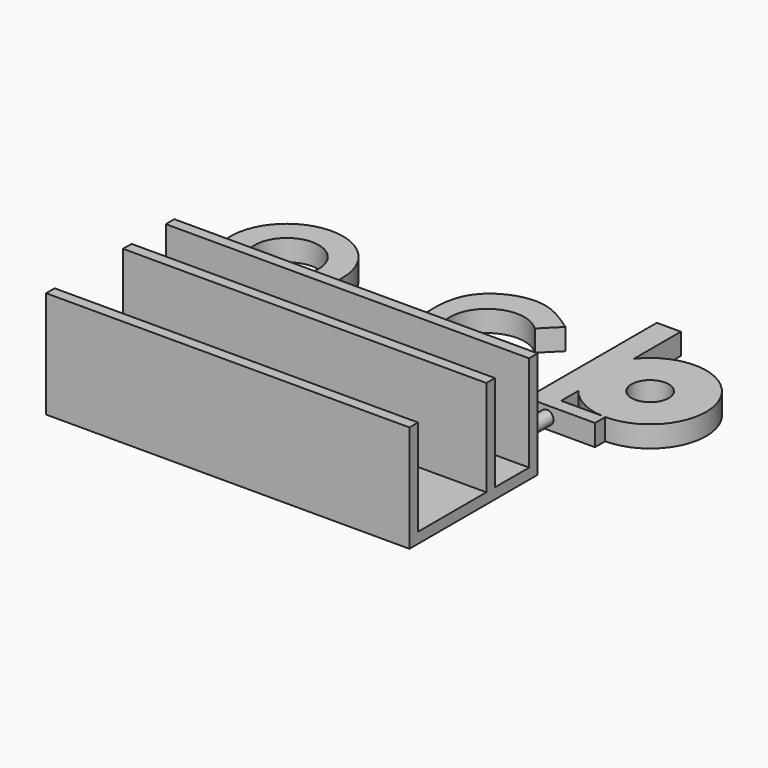
from build123d import *

# Parameters (mm, degrees)
F1_R      = 6
F2_DEPTH  = 4
F1_R_2    = 3.5
F0_R      = 7
F3_DEPTH  = 25
F5_DEPTH  = 4
F6_R      = 1.2123195681
F6_R_2    = 1.1427466474
F6_R_3    = 1.2541450495
F7_DEPTH  = 10
F9_W      = 68
F9_H      = 30
F10_DEPTH = 20
F11_W     = 68
F11_H     = 8
F11_H_2   = 16
F12_DEPTH = 18
F13_R     = 1.26
F14_DEPTH = 25


with BuildPart() as f2:
    # F1 (on Top) → F2 (new body)
    with BuildSketch(Plane.XY):
        with BuildLine():
            ThreePointArc((6, -8.6168439698), (9.3072552345, -4.8605555238), (10.5, 0))
            ThreePointArc((10.5, 0), (-9.3072552345, 4.8605555238), (6, -8.6168439698))
        make_face()
        Circle(F1_R, mode=Mode.SUBTRACT)
        with BuildLine():
            Line((10.5, -10.5), (10.5, 0))
            ThreePointArc((10.5, 0), (9.3072552345, -4.8605555238), (6, -8.6168439698))
            Line((6, -8.6168439698), (6, -10.5))
            Line((6, -10.5), (10.5, -10.5))
        make_face()
    extrude(amount=F2_DEPTH)



with BuildPart() as f2b:
    # F1 (on Top) → F2, piece 2 (new body)
    with BuildSketch(Plane.XY):
        with BuildLine():
            ThreePointArc((32.75, -5.1417409503), (40.3062430401, -6.4128776692), (44.5, 0))
            ThreePointArc((44.5, 0), (43.9671567276, 2.6787840266), (42.4497474683, 4.9497474683))
            ThreePointArc((42.4497474683, 4.9497474683), (32.4532674542, 4.8508237044), (32.75, -5.1417409503))
        make_face()
        with BuildLine():
            ThreePointArc((32.75, -5.1417409503), (32.4532674542, 4.8508237044), (42.4497474683, 4.9497474683))
            Line((42.4497474683, 4.9497474683), (45.6317279836, 8.1317279836))
            add(Edge.make_bspline(
                [(28.25, -10.5), (27.0400886154, -3.8399480871), (24.8960722969, 7.9619575442), (37.8802140743, 13.5938400363), (43.1156627298, 9.9046758889), (45.6317279836, 8.1317279836)],
                knots=[0, 0, 0, 0, 0.4021935112, 0.7127046345, 1, 1, 1, 1], degree=3))
            Line((28.25, -10.5), (32.75, -10.5))
            Line((32.75, -10.5), (32.75, -5.1417409503))
        make_face()
    extrude(amount=F2_DEPTH)

    # F0 (on Top) → F3 (cut)
    with BuildSketch(Plane.XY):
        with Locations((37.5, 0)):
            Circle(F0_R)
    extrude(amount=F3_DEPTH, mode=Mode.SUBTRACT)


with BuildPart() as f2c:
    # F1 (on Top) → F2, piece 3 (new body)
    with BuildSketch(Plane.XY):
        with BuildLine():
            Line((55.25, 17.5), (55.25, -10.5))
            Line((55.25, -10.5), (59.75, -10.5))
            Line((59.75, -10.5), (59.75, -6.4951905284))
            ThreePointArc((59.75, -6.4951905284), (57.5, 0), (59.75, 6.4951905284))
            Line((59.75, 6.4951905284), (59.75, 17.5))
            Line((59.75, 17.5), (55.25, 17.5))
        make_face()
        with BuildLine():
            ThreePointArc((59.75, 6.4951905284), (57.5, 0), (59.75, -6.4951905284))
            Line((59.75, -6.4951905284), (59.75, 6.4951905284))
        make_face()
        with BuildLine():
            Line((59.75, 6.4951905284), (59.75, -6.4951905284))
            ThreePointArc((59.75, -6.4951905284), (71.4369317712, -9.9215674165), (78.5, 0))
            ThreePointArc((78.5, 0), (71.4369317712, 9.9215674165), (59.75, 6.4951905284))
        make_face()
        with Locations((68, 0)):
            Circle(F1_R_2, mode=Mode.SUBTRACT)
    extrude(amount=F2_DEPTH)


with BuildPart() as f2_1:
    add(f2.part)

    add(f2b.part)  # F5 merges F2b

    add(f2c.part)  # F5 merges F2c
    # F4 (on Top) → F5 (join)
    with BuildSketch(Plane.XY):
        Polygon((28.25, -10.5), (10.5, -10.5), (6, -10.5), (0, -10.5), (0, -12.9), (68, -12.9), (68, -10.5), (59.75, -10.5), (55.25, -10.5), (32.75, -10.5), align=None)
        with BuildLine():
            Line((6, -10.5), (10.5, -10.5))
            Line((10.5, -10.5), (28.25, -10.5))
            Line((28.25, -10.5), (32.75, -10.5))
            Line((32.75, -10.5), (55.25, -10.5))
            Line((55.25, -10.5), (59.75, -10.5))
            Line((59.75, -10.5), (68, -10.5))
            ThreePointArc((68, -10.5), (67.7708712153, -10.4974997023), (67.5418515524, -10.49))
            Line((67.5418515524, -10.49), (0.4581484476, -10.49))
            ThreePointArc((0.4581484476, -10.49), (0.2291287847, -10.4974997023), (0, -10.5))
            Line((0, -10.5), (6, -10.5))
        make_face()
    extrude(amount=F5_DEPTH)

    # F6 (on face) → F7 (join)
    with BuildSketch(Plane.XZ.offset(12.9)):
        with Locations((9, 2)):
            Circle(F6_R)
        with Locations((34, 2)):
            Circle(F6_R_2)
        with Locations((59, 2)):
            Circle(F6_R_3)
    extrude(amount=F7_DEPTH)

    # F8: union 


with BuildPart() as f10:
    # F9 (on Top) → F10 (new body)
    with BuildSketch(Plane.XY):
        with Locations((32.9095590711, -39.9419295043)):
            Rectangle(F9_W, F9_H)
    extrude(amount=F10_DEPTH)

    # F11 (on face) → F12 (cut)
    with BuildSketch(Plane.XY.offset(20)):
        with Locations((32.9095590711, -30.9419295043)):
            Rectangle(F11_W, F11_H)
        with Locations((32.9095590711, -44.9419295043)):
            Rectangle(F11_W, F11_H_2)
    extrude(amount=-F12_DEPTH, mode=Mode.SUBTRACT)

    # F13 (on face) → F14 (cut)
    with BuildSketch(Plane.XY.offset(2)):
        with Locations((7.9095590711, -30.9419295043)):
            Circle(F13_R)
        with Locations((32.9095590711, -30.9419295043)):
            Circle(F13_R)
        with Locations((57.9095590711, -30.9419295043)):
            Circle(F13_R)
    extrude(amount=-F14_DEPTH, mode=Mode.SUBTRACT)


solid = Compound([f2_1.part, f10.part])
